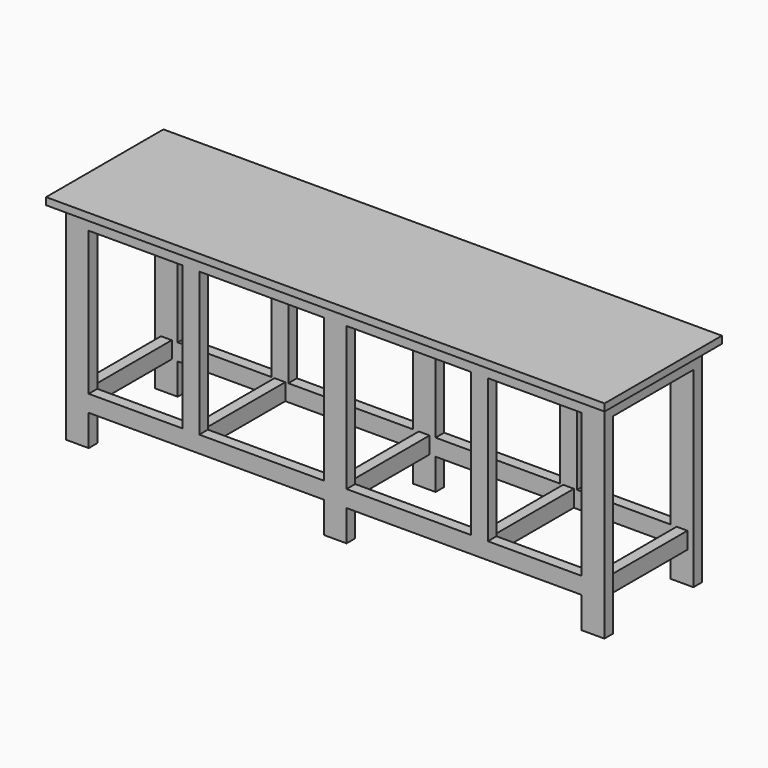
from build123d import *

# Parameters (mm, degrees)
F1_W      = 2334
F1_H      = 613
F2_DEPTH  = 30
F3_W      = 45
F3_H      = 420
F3_W_2    = 982.5
F3_H_2    = 45
F4_DEPTH  = 70
F5_DEPTH  = 870
F8_W      = 45
F8_H      = 420
F9_DEPTH  = 70
F10_DEPTH = 670
F11_DEPTH = 70


# Not quite as in the source:
# - a feature names something its author has since deleted; it is built from what else it names


with BuildPart() as f2:
    # F1 (on offset) → F2 (new body)
    with BuildSketch(Plane.XY.offset(900)):
        Rectangle(F1_W, F1_H)
    extrude(amount=-F2_DEPTH)

    # F3 (on face) → F4 (join)
    with BuildSketch(Plane(origin=(0, 0, 870), x_dir=(1, 0, 0), z_dir=(0, 0, -1))):
        with Locations((-1102.5, 0)):
            Rectangle(F3_W, F3_H)
        with Locations((1102.5, 0)):
            Rectangle(F3_W, F3_H)
        with Locations((-538.75, 232.5)):
            Rectangle(F3_W_2, F3_H_2)
        with Locations((-538.75, -232.5)):
            Rectangle(F3_W_2, F3_H_2)
        Polygon((47.5, 255), (-47.5, 255), (-47.5, 210), (-22.5, 210), (22.5, 210), (47.5, 210), align=None)
        with Locations((538.75, 232.5)):
            Rectangle(F3_W_2, F3_H_2)
        Polygon((22.5, 210), (-22.5, 210), (-22.5, -210), (22.5, -210), (22.5, -47.5), (22.5, 47.5), align=None)
        with Locations((538.75, -232.5)):
            Rectangle(F3_W_2, F3_H_2)
    extrude(amount=F4_DEPTH)

    # F3 (on face) → F5 (join)
    with BuildSketch(Plane(origin=(0, 0, 870), x_dir=(1, 0, 0), z_dir=(0, 0, -1))):
        Polygon((-1030, 255), (-1125, 255), (-1125, 210), (-1080, 210), (-1030, 210), align=None)
        Polygon((47.5, 255), (-47.5, 255), (-47.5, 210), (-22.5, 210), (22.5, 210), (47.5, 210), align=None)
        Polygon((-1080, -210), (-1125, -210), (-1125, -255), (-1030, -255), (-1030, -210), align=None)
        Polygon((1125, 255), (1030, 255), (1030, 210), (1080, 210), (1125, 210), align=None)
        Polygon((22.5, -210), (-22.5, -210), (-47.5, -210), (-47.5, -255), (47.5, -255), (47.5, -210), align=None)
        Polygon((1125, -255), (1125, -210), (1080, -210), (1030, -210), (1030, -255), align=None)
    extrude(amount=F5_DEPTH)

    # F8 (on offset) → F9 (join)
    with BuildSketch(Plane.XY.offset(130)):
        Polygon((-638, 210), (-638, 255), (-1100, 255), (-1100, -255), (-638, -255), (-638, -210), (-1055, -210), (-1055, 210), align=None)
        Polygon((568, 210), (568, 255), (-568, 255), (-568, 210), (-22.5, 210), (22.5, 210), align=None)
        Polygon((-568, -255), (568, -255), (568, -210), (22.5, -210), (-22.5, -210), (-568, -210), align=None)
        Rectangle(F8_W, F8_H)
        Polygon((1100, -255), (1100, 255), (638, 255), (638, 210), (1055, 210), (1055, -210), (638, -210), (638, -255), align=None)
    extrude(amount=F9_DEPTH)

    # F8 (on offset) → F10 (join, through all)
    with BuildSketch(Plane.XY.offset(130)):
        Polygon((-638, -255), (-568, -255), (-568, -210), (-580.5, -210), (-625.5, -210), (-638, -210), align=None)
        Polygon((-568, 210), (-568, 255), (-638, 255), (-638, 210), (-625.5, 210), (-580.5, 210), align=None)
        Polygon((638, 210), (638, 255), (568, 255), (568, 210), (580.5, 210), (625.5, 210), align=None)
        Polygon((568, -255), (638, -255), (638, -210), (625.5, -210), (580.5, -210), (568, -210), align=None)
    extrude(amount=F10_DEPTH)

    # F8 (on offset) → F11 (join)
    with BuildSketch(Plane.XY.offset(130)):
        with Locations((-603, 0)):
            Rectangle(F8_W, F8_H)
        with Locations((603, 0)):
            Rectangle(F8_W, F8_H)
    extrude(amount=F11_DEPTH)


solid = f2.part
